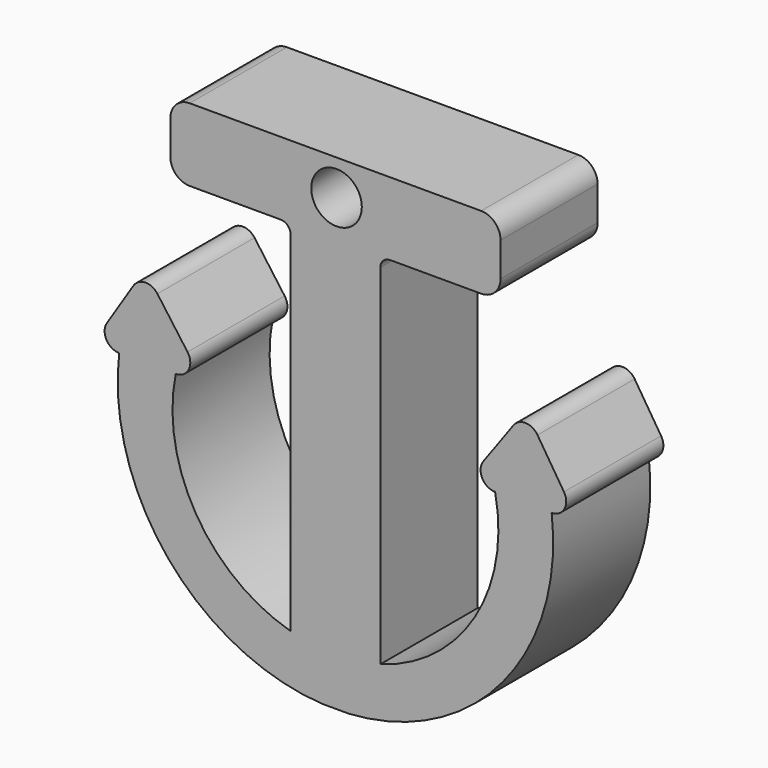
from build123d import *

# Parameters (mm, degrees)
F0_W     = 25.4
F0_H     = 25.4
F1_DEPTH = 6.35
F3_DEPTH = 25.4
F4_R     = 1.3225172329
F5_DEPTH = 25.4


# Not quite as in the source:
# - a feature names something its author has since deleted; it is built from what else it names


with BuildPart() as f1:
    # F0 (on Front) → F1 (new body)
    with BuildSketch(Plane.XZ):
        with Locations((12.7, 12.7)):
            Rectangle(F0_W, F0_H)
    extrude(amount=F1_DEPTH)

    # F2 (on face) → F3 (cut)
    with BuildSketch(Plane.XZ.offset(6.35)):
        with BuildLine():
            ThreePointArc((4.347079063, 12.7), (5.4149768535, 6.5815794315), (10.3514468814, 2.8123965482))
            Line((10.3514468814, 2.8123965482), (10.3514468814, 21.082))
            ThreePointArc((10.3514468814, 21.082), (10.2026571262, 21.4412102448), (9.8434468814, 21.59))
            Line((9.8434468814, 21.59), (5.08, 21.59))
            ThreePointArc((5.08, 21.59), (4.3615795103, 21.8875795103), (4.064, 22.606))
            Line((4.064, 22.606), (4.064, 24.384))
            ThreePointArc((4.064, 24.384), (4.3615795103, 25.1024204897), (5.08, 25.4))
            Line((5.08, 25.4), (0, 25.4))
            Line((0, 25.4), (0, 0))
            Line((0, 0), (11.9920649295, 0))
            ThreePointArc((11.9920649295, 0), (3.957639074, 4.0680963279), (1.3902190546, 12.7))
            ThreePointArc((1.3902190546, 12.7), (0.7220113765, 13.0957453087), (0.7478720811, 13.8719199503))
            Line((0.7478720811, 13.8719199503), (2.1310466878, 16.0393626953))
            ThreePointArc((2.1310466878, 16.0393626953), (2.7505395089, 16.3910999432), (3.390007158, 16.0771388424))
            Line((3.390007158, 16.0771388424), (4.9636925598, 13.9096960974))
            ThreePointArc((4.9636925598, 13.9096960974), (5.025970964, 13.1159511785), (4.347079063, 12.7))
        make_face()
        with BuildLine():
            Line((25.4, 25.4), (20.32, 25.4))
            ThreePointArc((20.32, 25.4), (21.0384204897, 25.1024204897), (21.336, 24.384))
            Line((21.336, 24.384), (21.336, 22.606))
            ThreePointArc((21.336, 22.606), (21.0384204897, 21.8875795103), (20.32, 21.59))
            Line((20.32, 21.59), (15.5565531186, 21.59))
            ThreePointArc((15.5565531186, 21.59), (15.1973428738, 21.4412102448), (15.0485531186, 21.082))
            Line((15.0485531186, 21.082), (15.0485531186, 15.5096852131))
            Line((15.0485531186, 15.5096852131), (15.0485531186, 2.8123965482))
            ThreePointArc((15.0485531186, 2.8123965482), (19.9850231465, 6.5815794315), (21.052920937, 12.7))
            ThreePointArc((21.052920937, 12.7), (20.374029036, 13.1159511785), (20.4363074402, 13.9096960974))
            Line((20.4363074402, 13.9096960974), (22.009992842, 16.0771388424))
            ThreePointArc((22.009992842, 16.0771388424), (22.6494604911, 16.3910999432), (23.2689533122, 16.0393626953))
            Line((23.2689533122, 16.0393626953), (24.6521279189, 13.8719199503))
            ThreePointArc((24.6521279189, 13.8719199503), (24.6779886235, 13.0957453087), (24.0097809454, 12.7))
            ThreePointArc((24.0097809454, 12.7), (21.442360926, 4.0680963279), (13.4079350705, 0))
            Line((13.4079350705, 0), (25.4, 0))
            Line((25.4, 0), (25.4, 25.4))
        make_face()
    extrude(amount=-F3_DEPTH, mode=Mode.SUBTRACT)

    # F4 (on Front) → F5 (cut)
    with BuildSketch(Plane.XZ):
        with Locations((12.7565525472, 23.5501565039)):
            Circle(F4_R)
    extrude(amount=F5_DEPTH, mode=Mode.SUBTRACT)


solid = f1.part
